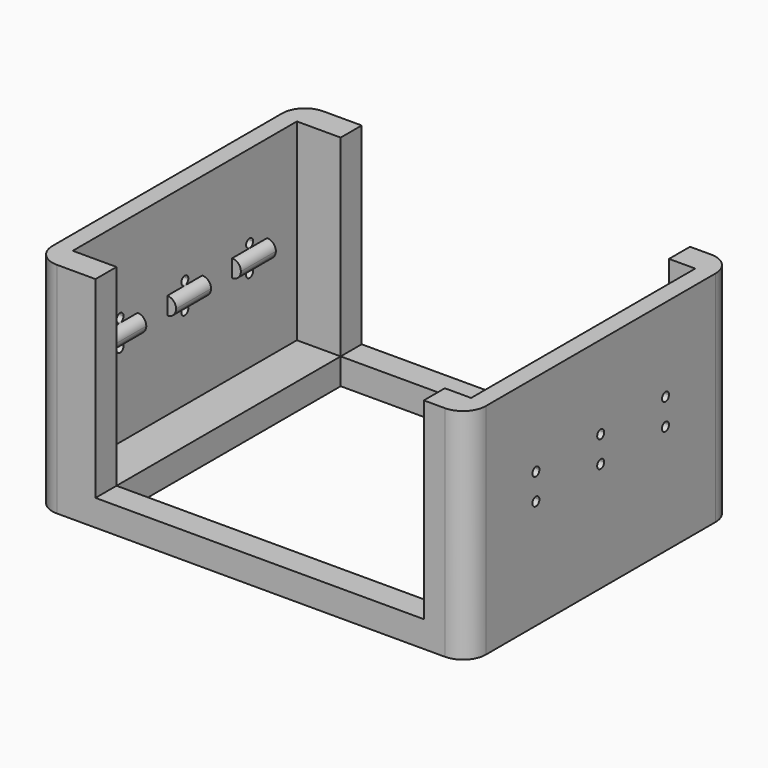
from build123d import *

# Parameters (mm, degrees)
F0_W      = 2
F0_H      = 32
F0_H_2    = 3
F0_W_2    = 5
F1_DEPTH  = 25
F0_W_3    = 3
F0_W_4    = 37.5
F2_DEPTH  = 3
F3_R      = 2.6
F6_DEPTH  = 1
F7_R      = 0.99999
F10_DEPTH = 1
F11_R     = 0.99999
F12_DEPTH = 5
F13_DEPTH = 5


# Not quite as in the source:
# - a fillet or chamfer is up to 0.001 mm smaller than in the source, because OpenCascade refuses the exact size
# - a feature names something its author has since deleted; it is built from what else it names


with BuildPart() as f1:
    # F0 (on Top) → F1 (new body)
    with BuildSketch(Plane.XY):
        with Locations((-23.75, 0)):
            Rectangle(F0_W, F0_H)
        with Locations((-23.75, 17.5)):
            Rectangle(F0_W, F0_H_2)
        with Locations((-23.75, -17.5)):
            Rectangle(F0_W, F0_H_2)
        with Locations((-20.25, 17.5)):
            Rectangle(F0_W_2, F0_H_2)
        with Locations((-20.25, -17.5)):
            Rectangle(F0_W_2, F0_H_2)
    extrude(amount=F1_DEPTH)



with BuildPart() as f1b:
    # F0 (on Top) → F1, piece 2 (new body)
    with BuildSketch(Plane.XY):
        with Locations((21.25, -17.5)):
            Rectangle(F0_W_3, F0_H_2)
        with Locations((23.75, -17.5)):
            Rectangle(F0_W, F0_H_2)
        with Locations((23.75, 0)):
            Rectangle(F0_W, F0_H)
        with Locations((23.75, 17.5)):
            Rectangle(F0_W, F0_H_2)
        with Locations((21.25, 17.5)):
            Rectangle(F0_W_3, F0_H_2)
    extrude(amount=F1_DEPTH)


with BuildPart() as f1_1:
    add(f1.part)

    add(f1b.part)  # F2 merges F1b
    # F0 (on Top) → F2 (join)
    with BuildSketch(Plane.XY):
        with Locations((21.25, 0)):
            Rectangle(F0_W_3, F0_H)
        with Locations((1, 17.5)):
            Rectangle(F0_W_4, F0_H_2)
        with Locations((-20.25, 0)):
            Rectangle(F0_W_2, F0_H)
        with Locations((1, -17.5)):
            Rectangle(F0_W_4, F0_H_2)
    extrude(amount=F2_DEPTH)

    # F3
    f3_edges = [f1_1.edges().sort_by_distance(p)[0] for p in [
        (-24.75, 19, 12.5),
        (24.75, 19, 12.5),
        (24.75, -19, 12.5),
        (-24.75, -19, 12.5),
    ]]
    fillet(f3_edges, radius=F3_R)

    # F5 (on face) → F6 (join)
    with BuildSketch(Plane.YZ.offset(22.75)):
        Polygon((-11.75, 15), (-11.75, 13), (-9.25, 13), (-6.75, 13), (-6.75, 15), (-9.25, 15), align=None)
        Polygon((-2.5, 15), (-2.5, 13), (0, 13), (2.5, 13), (2.5, 15), (0, 15), align=None)
        Polygon((6.75, 15), (6.75, 13), (9.25, 13), (11.75, 13), (11.75, 15), (9.25, 15), align=None)
    extrude(amount=-F6_DEPTH)

    # F7 (radius 1 in the source; OpenCascade refuses exactly that, so slightly less here)
    f7_edges = [f1_1.edges().sort_by_distance(p)[0] for p in [
        (21.75, -9.25, 15),
        (21.75, -9.25, 13),
        (21.75, 0, 15),
        (21.75, 0, 13),
        (21.75, 9.25, 13),
        (21.75, 9.25, 15),
    ]]
    fillet(f7_edges, radius=F7_R)

    # F9 (on face) → F10 (join)
    with BuildSketch(Plane.YZ.offset(-22.75)):
        Polygon((-11.75, 15), (-11.75, 13), (-9.25, 13), (-6.75, 13), (-6.75, 15), (-9.25, 15), align=None)
        Polygon((-2.5, 15), (-2.5, 13), (0, 13), (2.5, 13), (2.5, 15), (0, 15), align=None)
        Polygon((6.75, 15), (6.75, 13), (9.25, 13), (11.75, 13), (11.75, 15), (9.25, 15), align=None)
    extrude(amount=F10_DEPTH)

    # F11 (radius 1 in the source; OpenCascade refuses exactly that, so slightly less here)
    f11_edges = [f1_1.edges().sort_by_distance(p)[0] for p in [
        (-21.75, -9.25, 15),
        (-21.75, -9.25, 13),
        (-21.75, 0, 15),
        (-21.75, 9.25, 15),
        (-21.75, 0, 13),
        (-21.75, 9.25, 13),
    ]]
    fillet(f11_edges, radius=F11_R)

    # F5 (on face) → F12 (cut)
    with BuildSketch(Plane.YZ.offset(22.75)):
        with BuildLine():
            ThreePointArc((-8.75, 15.5), (-9.6035533906, 15.8535533906), (-9.25, 15))
            ThreePointArc((-9.25, 15), (-8.8964466094, 15.1464466094), (-8.75, 15.5))
        make_face()
        with BuildLine():
            ThreePointArc((0.5, 15.5), (-0.3535533906, 15.8535533906), (0, 15))
            ThreePointArc((0, 15), (0.3535533906, 15.1464466094), (0.5, 15.5))
        make_face()
        with BuildLine():
            ThreePointArc((9.75, 15.5), (8.8964466094, 15.8535533906), (9.25, 15))
            ThreePointArc((9.25, 15), (9.6035533906, 15.1464466094), (9.75, 15.5))
        make_face()
        with BuildLine():
            ThreePointArc((9.75, 12.5), (9.6035533906, 12.8535533906), (9.25, 13))
            ThreePointArc((9.25, 13), (8.8964466094, 12.1464466094), (9.75, 12.5))
        make_face()
        with BuildLine():
            ThreePointArc((0.5, 12.5), (0.3535533906, 12.8535533906), (0, 13))
            ThreePointArc((0, 13), (-0.3535533906, 12.1464466094), (0.5, 12.5))
        make_face()
        with BuildLine():
            ThreePointArc((-8.75, 12.5), (-8.8964466094, 12.8535533906), (-9.25, 13))
            ThreePointArc((-9.25, 13), (-9.6035533906, 12.1464466094), (-8.75, 12.5))
        make_face()
    extrude(amount=F12_DEPTH, mode=Mode.SUBTRACT)

    # F9 (on face) → F13 (cut)
    with BuildSketch(Plane.YZ.offset(-22.75)):
        with BuildLine():
            ThreePointArc((-8.75, 15.5), (-9.6035533906, 15.8535533906), (-9.25, 15))
            ThreePointArc((-9.25, 15), (-8.8964466094, 15.1464466094), (-8.75, 15.5))
        make_face()
        with BuildLine():
            ThreePointArc((0.5, 15.5), (-0.3535533906, 15.8535533906), (0, 15))
            ThreePointArc((0, 15), (0.3535533906, 15.1464466094), (0.5, 15.5))
        make_face()
        with BuildLine():
            ThreePointArc((9.75, 15.5), (8.8964466094, 15.8535533906), (9.25, 15))
            ThreePointArc((9.25, 15), (9.6035533906, 15.1464466094), (9.75, 15.5))
        make_face()
        with BuildLine():
            ThreePointArc((9.75, 12.5), (9.6035533906, 12.8535533906), (9.25, 13))
            ThreePointArc((9.25, 13), (8.8964466094, 12.1464466094), (9.75, 12.5))
        make_face()
        with BuildLine():
            ThreePointArc((0.5, 12.5), (0.3535533906, 12.8535533906), (0, 13))
            ThreePointArc((0, 13), (-0.3535533906, 12.1464466094), (0.5, 12.5))
        make_face()
        with BuildLine():
            ThreePointArc((-8.75, 12.5), (-8.8964466094, 12.8535533906), (-9.25, 13))
            ThreePointArc((-9.25, 13), (-9.6035533906, 12.1464466094), (-8.75, 12.5))
        make_face()
    extrude(amount=-F13_DEPTH, mode=Mode.SUBTRACT)


solid = f1_1.part
